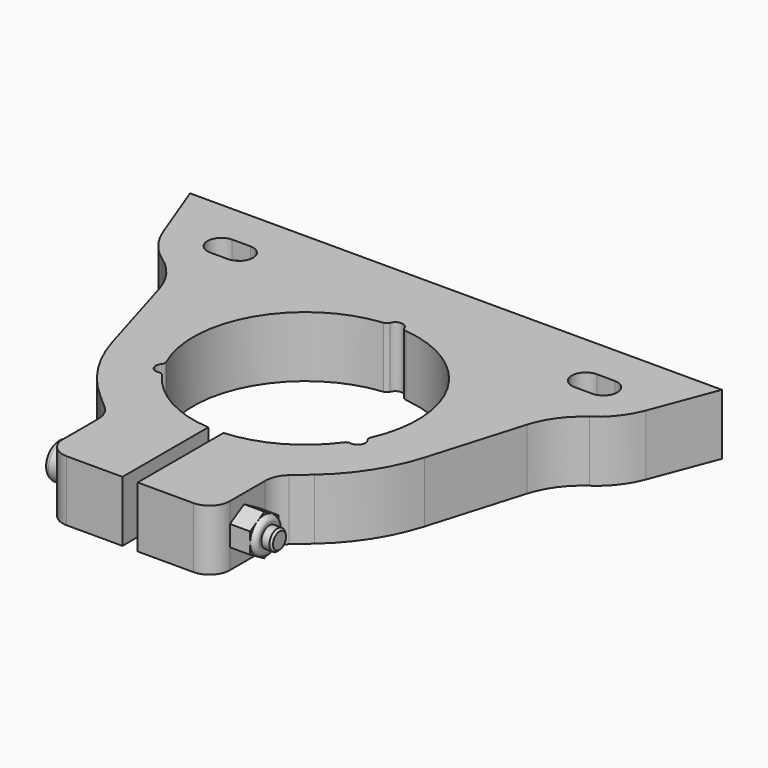
from build123d import *

# Parameters (mm, degrees)
F1_DEPTH  = 12
F2_R      = 5
F3_R      = 2
F4_DEPTH  = 69.001
F5_R      = 4
F6_R      = 3.5
F7_DEPTH  = 3.8
F8_R      = 2
F9_DEPTH  = 40
F10_R     = 2
F11_DEPTH = 4
F12_R     = 3.5
F12_R_2   = 2
F13_DEPTH = 1
F14_R     = 0.99999
F15_SIZE  = 0.4
F17_DEPTH = 3
F18_R     = 1
F19_R     = 2
F19_R_2   = 2.7749854476
F20_DEPTH = 12
F21_R     = 1.5
F22_DEPTH = 25
F23_R     = 1


# Not quite as in the source:
# - a fillet or chamfer is up to 0.001 mm smaller than in the source, because OpenCascade refuses the exact size


with BuildPart() as f1:
    # F0 (on Top) → F1 (new body)
    with BuildSketch(Plane.XY):
        with BuildLine():
            Line((52.5, 0), (-52.5, 0))
            Line((-52.5, 0), (-47.6682177495, -12.7529115916))
            ThreePointArc((-47.6682177495, -12.7529115916), (-45.4487126417, -16.689553935), (-42.1574376197, -19.7864660409))
            ThreePointArc((-42.1574376197, -19.7864660409), (-38.5340554499, -23.3236951077), (-36.2940938248, -27.8650010584))
            Line((-36.2940938248, -27.8650010584), (-30.8201520188, -46.3009960956))
            ThreePointArc((-30.8201520188, -46.3009960956), (-27.0602921577, -54.5098124511), (-21.1662026167, -61.3494703824))
            Line((-21.1662026167, -61.3494703824), (-16.5, -65.4307906954))
            Line((-16.5, -65.4307906954), (-16.5, -80.4307906954))
            Line((-16.5, -80.4307906954), (-1.5, -80.4307906954))
            Line((-1.5, -80.4307906954), (-1.5, -59.2491515674))
            ThreePointArc((-1.5, -59.2491515674), (0, -15), (1.5, -59.2491515674))
            Line((1.5, -59.2491515674), (1.5, -80.4307906954))
            Line((1.5, -80.4307906954), (16.5, -80.4307906954))
            Line((16.5, -80.4307906954), (16.5, -65.4307906954))
            Line((16.5, -65.4307906954), (21.1662026167, -61.3494703824))
            ThreePointArc((21.1662026167, -61.3494703824), (27.0602921577, -54.5098124511), (30.8201520188, -46.3009960956))
            Line((30.8201520188, -46.3009960956), (36.2940938248, -27.8650010584))
            ThreePointArc((36.2940938248, -27.8650010584), (38.5340554499, -23.3236951077), (42.1574376197, -19.7864660409))
            ThreePointArc((42.1574376197, -19.7864660409), (45.4487126417, -16.689553935), (47.6682177495, -12.7529115916))
            Line((47.6682177495, -12.7529115916), (52.5, 0))
        make_face()
        with BuildLine():
            Line((-34.2147789885, -13.5), (-37.6424851382, -13.5))
            ThreePointArc((-37.6424851382, -13.5), (-40.4638530749, -10.8213679366), (-37.7852210115, -8))
            Line((-37.7852210115, -8), (-34.2147789885, -8))
            ThreePointArc((-34.2147789885, -8), (-31.4647789885, -10.75), (-34.2147789885, -13.5))
        make_face(mode=Mode.SUBTRACT)
        with BuildLine():
            ThreePointArc((37.7852210115, -8), (40.4638530749, -10.8213679366), (37.6424851382, -13.5))
            Line((37.6424851382, -13.5), (34.2147789885, -13.5))
            ThreePointArc((34.2147789885, -13.5), (31.4647789885, -10.75), (34.2147789885, -8))
            Line((34.2147789885, -8), (37.7852210115, -8))
        make_face(mode=Mode.SUBTRACT)
    extrude(amount=F1_DEPTH)

    # F2
    f2_edges = [f1.edges().sort_by_distance(p)[0] for p in [
        (-16.5, -65.430791, 6),
        (16.5, -65.430791, 6),
    ]]
    fillet(f2_edges, radius=F2_R)

    # F3 (on face) → F4 (cut, through all)
    with BuildSketch(Plane(origin=(-16.5, 0, 0), x_dir=(0, -1, 0), z_dir=(-1, 0, 0))):
        with Locations((72.9307906954, 6)):
            Circle(F3_R)
    extrude(amount=-F4_DEPTH, mode=Mode.SUBTRACT)

    # F5
    f5_edges = [f1.edges().sort_by_distance(p)[0] for p in [
        (-16.5, -80.430791, 6),
        (16.5, -80.430791, 6),
    ]]
    fillet(f5_edges, radius=F5_R)

    # F19 (on face) → F20 (cut)
    with BuildSketch(Plane(origin=(0, 0, 0), x_dir=(-1, 0, 0), z_dir=(0, 1, 0))):
        with Locations((-36, 6)):
            Circle(F19_R)
        with Locations((36, 6)):
            Circle(F19_R_2)
    extrude(amount=-F20_DEPTH, mode=Mode.SUBTRACT)

    # F21 (on face) → F22 (cut)
    with BuildSketch(Plane.XY.offset(12)):
        with Locations((0, -15)):
            Circle(F21_R)
        with Locations((-19.1824626938, -48.225)):
            Circle(F21_R)
        with Locations((19.1824626938, -48.225)):
            Circle(F21_R)
    extrude(amount=-F22_DEPTH, mode=Mode.SUBTRACT)

    # F23
    f23_edges = [f1.edges().sort_by_distance(p)[0] for p in [
        (1.49914, -15.05079, 6),
        (-1.49914, -15.05079, 6),
        (-19.888047, -46.901312, 6),
        (-18.388907, -49.497898, 6),
        (18.388907, -49.497898, 6),
        (19.888047, -46.901312, 6),
    ]]
    fillet(f23_edges, radius=F23_R)


with BuildPart() as f7:
    # F6 (on face) → F7 (new body)
    with BuildSketch(Plane(origin=(-16.5, 0, 0), x_dir=(0, -1, 0), z_dir=(-1, 0, 0))):
        with Locations((72.9307906954, 6)):
            Circle(F6_R)
    extrude(amount=F7_DEPTH)

    # F8 (on face) → F9 (join)
    with BuildSketch(Plane.YZ.offset(-16.5)):
        with Locations((-72.9307906954, 6)):
            Circle(F8_R)
    extrude(amount=F9_DEPTH)

    # F15
    f15_edges = [f7.edges().sort_by_distance(p)[0] for p in [
        (23.5, -74.930791, 6),
    ]]
    chamfer(f15_edges, length=F15_SIZE)

    # F16 (on face) → F17 (cut)
    with BuildSketch(Plane(origin=(-20.3, 0, 0), x_dir=(0, -1, 0), z_dir=(-1, 0, 0))):
        Polygon((73.9905514021, 3.9481129227), (75.2376573834, 5.8918361553), (74.1778966767, 7.9437232326), (71.8710299887, 8.0518870773), (70.6239240075, 6.1081638447), (71.6836847142, 4.0562767674), align=None)
    extrude(amount=-F17_DEPTH, mode=Mode.SUBTRACT)

    # F18
    f18_edges = [f7.edges().sort_by_distance(p)[0] for p in [
        (-20.3, -69.430791, 6),
    ]]
    fillet(f18_edges, radius=F18_R)


with BuildPart() as f11:
    # F10 (on face) → F11 (new body)
    with BuildSketch(Plane.YZ.offset(16.5)):
        Polygon((-76.4373237522, 3.9906321255), (-72.9438935989, 1.9585693564), (-69.4373605421, 3.9679372309), (-69.4242576387, 8.0093678745), (-72.9176877919, 10.0414306436), (-76.4242208487, 8.0320627691), align=None)
        with Locations((-72.9307906954, 6)):
            Circle(F10_R, mode=Mode.SUBTRACT)
    extrude(amount=F11_DEPTH)

    # F12 (on face) → F13 (join)
    with BuildSketch(Plane.YZ.offset(20.5)):
        with Locations((-72.9307906954, 6)):
            Circle(F12_R)
        with Locations((-72.9307906954, 6)):
            Circle(F12_R_2, mode=Mode.SUBTRACT)
    extrude(amount=F13_DEPTH)

    # F14 (radius 1 in the source; OpenCascade refuses exactly that, so slightly less here)
    f14_edges = [f11.edges().sort_by_distance(p)[0] for p in [
        (21.5, -76.430791, 6),
    ]]
    fillet(f14_edges, radius=F14_R)


solid = Compound([f1.part, f7.part, f11.part])
